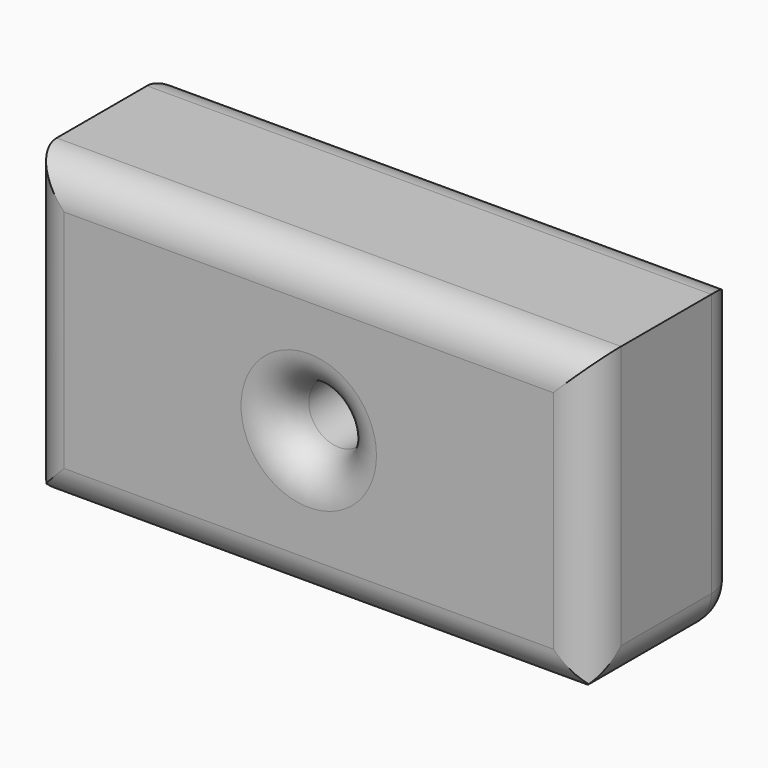
from build123d import *

# Parameters (mm, degrees)
F0_W         = 75
F0_H         = 40
F1_DEPTH     = 25
F2_R         = 4
F3_DEPTH     = 25
F4_R         = 5
F5_T1_DEPTH  = 27.5
F5_T3_DEPTH  = 65
F5_T5_DEPTH  = 47.5
F5_T7_DEPTH  = 100
F5_S11_W     = 5.1
F5_S11_H     = 5.1
F5_T12_DEPTH = 5.1
F5_S17_W     = 5.1
F5_S17_H     = 5.1
F5_T18_DEPTH = 5.1


# Not quite as in the source:
# - a fillet or chamfer that OpenCascade refuses, or shapes differently, is made with other operations: its cross-section is extruded or revolved along the edge and cut away or added


with BuildPart() as f1:
    # F0 (on Front) → F1 (new body)
    with BuildSketch(Plane.XZ):
        Rectangle(F0_W, F0_H)
    extrude(amount=F1_DEPTH)

    # F2 (on face) → F3 (cut)
    with BuildSketch(Plane.XZ.offset(25)):
        Circle(F2_R)
    extrude(amount=-F3_DEPTH, mode=Mode.SUBTRACT)

    # F4
    f4_edges = [f1.edges().sort_by_distance(p)[0] for p in [
        (0, -25, 20),
        (-37.5, -25, 0),
        (0, -25, -20),
        (37.5, -25, 0),
    ]]
    fillet(f4_edges, radius=F4_R)

    # F5: fillet of radius 5 on 8 edges, made by hand

    # F5_s2 → F5_t1 (cut)
    with BuildSketch(Plane.XZ.offset(5)):
        with BuildLine():
            ThreePointArc((-32.5, -20), (-36.0355339059, -18.5355339059), (-37.5, -15))
            Line((-37.5, -15), (-37.5, -20))
            Line((-37.5, -20), (-32.5, -20))
        make_face()
        with BuildLine():
            ThreePointArc((37.5, -15), (36.0355339059, -18.5355339059), (32.5, -20))
            Line((32.5, -20), (37.5, -20))
            Line((37.5, -20), (37.5, -15))
        make_face()
    extrude(amount=F5_T1_DEPTH, mode=Mode.SUBTRACT)

    # F5_s4 → F5_t3 (cut)
    with BuildSketch(Plane.YZ.offset(-32.5)):
        with BuildLine():
            ThreePointArc((-5, -20), (-1.4644660941, -18.5355339059), (0, -15))
            Line((0, -15), (0, -20))
            Line((0, -20), (-5, -20))
        make_face()
    extrude(amount=F5_T3_DEPTH, mode=Mode.SUBTRACT)

    # F5_s6 → F5_t5 (cut)
    with BuildSketch(Plane.XY.offset(-15)):
        with BuildLine():
            ThreePointArc((37.5, -5), (36.0355339059, -1.4644660941), (32.5, 0))
            Line((32.5, 0), (37.5, 0))
            Line((37.5, 0), (37.5, -5))
        make_face()
        with BuildLine():
            ThreePointArc((-32.5, 0), (-36.0355339059, -1.4644660941), (-37.5, -5))
            Line((-37.5, -5), (-37.5, 0))
            Line((-37.5, 0), (-32.5, 0))
        make_face()
    extrude(amount=F5_T5_DEPTH, mode=Mode.SUBTRACT)

    # F5_s8 → F5_t7 (cut)
    with BuildSketch(Plane.YZ.offset(-50)):
        with BuildLine():
            ThreePointArc((0, 15), (-1.4644660941, 18.5355339059), (-5, 20))
            Line((-5, 20), (0, 20))
            Line((0, 20), (0, 15))
        make_face()
    extrude(amount=F5_T7_DEPTH, mode=Mode.SUBTRACT)


with BuildPart() as f5_tool10:
    # F5_s11 → F5_t12 (new body)
    with BuildSketch(Plane.XY.offset(-15)):
        with Locations((-35.05, -2.45)):
            Rectangle(F5_S11_W, F5_S11_H)
    extrude(amount=-F5_T12_DEPTH)

    # F5_s13 → F5_t14 (revolve, cut)
    with BuildSketch(Plane(origin=(-32.5, -5, -15), x_dir=(0.7071067812, -0.7071067812, 0), z_dir=(0.7071067812, 0.7071067812, 0))):
        with BuildLine():
            ThreePointArc((0, -5), (5, 0), (0, 5))
            Line((0, 5), (0, -5))
        make_face()
    revolve(axis=Axis((-32.5, -5, -15), (0, 0, -1)), mode=Mode.SUBTRACT)


with BuildPart() as f1_1:
    add(f1.part)

    # F5_t9: cut F5_tool10
    add(f5_tool10.part, mode=Mode.SUBTRACT)


with BuildPart() as f5_tool16:
    # F5_s17 → F5_t18 (new body)
    with BuildSketch(Plane.YZ.offset(32.5)):
        with Locations((-2.45, -17.55)):
            Rectangle(F5_S17_W, F5_S17_H)
    extrude(amount=F5_T18_DEPTH)

    # F5_s19 → F5_t20 (revolve, cut)
    with BuildSketch(Plane(origin=(32.5, -5, -15), x_dir=(0, -0.7071067812, 0.7071067812), z_dir=(0, 0.7071067812, 0.7071067812))):
        with BuildLine():
            ThreePointArc((0, -5), (5, 0), (0, 5))
            Line((0, 5), (0, -5))
        make_face()
    revolve(axis=Axis((32.5, -5, -15), (1, 0, 0)), mode=Mode.SUBTRACT)


with BuildPart() as f1_2:
    add(f1_1.part)

    # F5_t15: cut F5_tool16
    add(f5_tool16.part, mode=Mode.SUBTRACT)

    # F5_s21 → F5_t22 (revolve, cut)
    with BuildSketch(Plane.XY):
        with BuildLine():
            ThreePointArc((9, -25), (5.4644660941, -23.5355339059), (4, -20))
            Line((4, -20), (4, -25))
            Line((4, -25), (9, -25))
        make_face()
    revolve(axis=Axis((0, -25, 0), (0, -1, 0)), mode=Mode.SUBTRACT)


solid = f1_2.part
